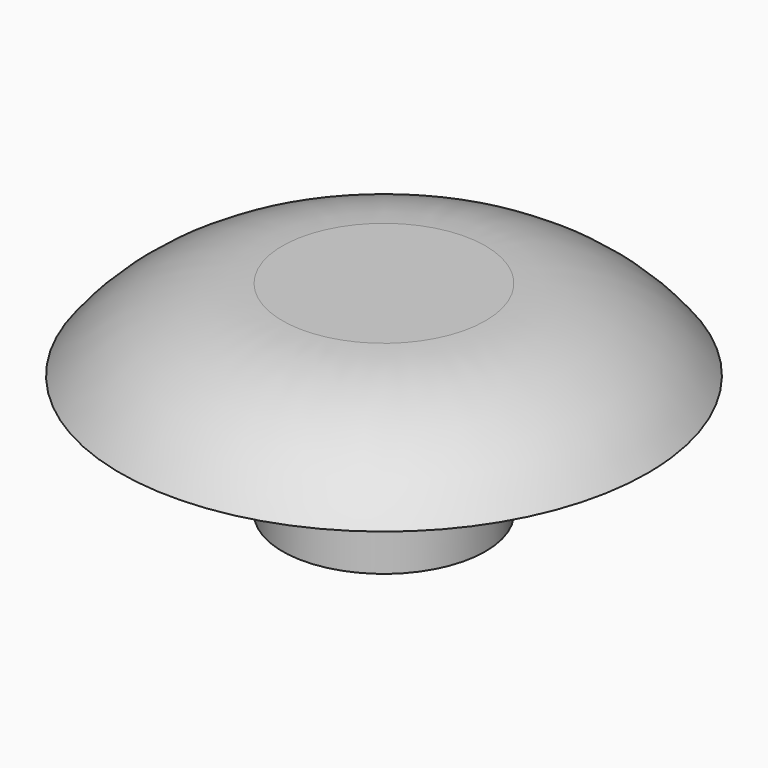
from build123d import *

# Parameters (mm, degrees)
F0_R     = 7.5
F1_DEPTH = 5
F2_R     = 4.99999
F3_W     = 2.6
F3_H     = 2.6
F4_DEPTH = 2.5
F5_R     = 7.5
F5_R_2   = 2.5
F6_DEPTH = 3


# Not quite as in the source:
# - a fillet or chamfer is up to 0.001 mm smaller than in the source, because OpenCascade refuses the exact size


with BuildPart() as f1:
    # F0 (on Top) → F1 (new body)
    with BuildSketch(Plane.XY):
        Circle(F0_R)
    extrude(amount=F1_DEPTH)

    # F2 (radius 5 in the source; OpenCascade refuses exactly that, so slightly less here)
    f2_edges = [f1.edges().sort_by_distance(p)[0] for p in [
        (-7.5, 0, 5),
    ]]
    fillet(f2_edges, radius=F2_R)

    # F3 (on face) → F4 (cut)
    with BuildSketch(Plane(origin=(0, 0, 0), x_dir=(1, 0, 0), z_dir=(0, 0, -1))):
        Rectangle(F3_W, F3_H)
    extrude(amount=-F4_DEPTH, mode=Mode.SUBTRACT)

    # F5 (on face) → F6 (cut)
    with BuildSketch(Plane(origin=(0, 0, 0), x_dir=(1, 0, 0), z_dir=(0, 0, -1))):
        Circle(F5_R)
        Circle(F5_R_2, mode=Mode.SUBTRACT)
    extrude(amount=-F6_DEPTH, mode=Mode.SUBTRACT)


solid = f1.part
